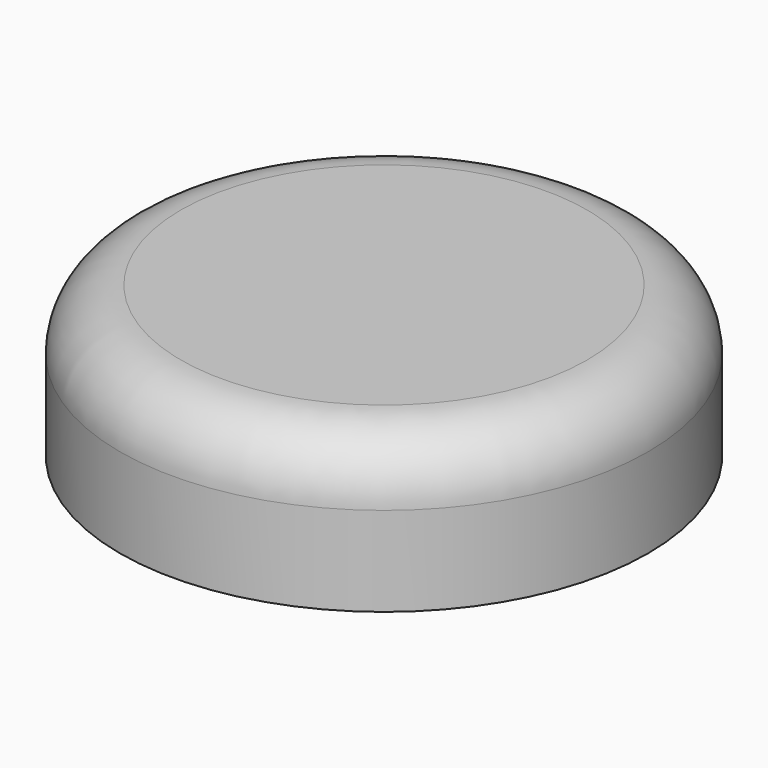
from build123d import *

# Parameters (mm, degrees)
F0_R     = 6.5
F1_DEPTH = 3.7
F2_R     = 1.5


# Not quite as in the source:
# - a feature of the source that left no trace in its solid (it failed there, or was rolled back) is left out


with BuildPart() as f1:
    # F0 (on Top) → F1 (new body)
    with BuildSketch(Plane.XY):
        Circle(F0_R)
    extrude(amount=F1_DEPTH)

    # F2
    f2_edges = [f1.edges().sort_by_distance(p)[0] for p in [
        (-6.5, 0, 3.7),
    ]]
    fillet(f2_edges, radius=F2_R)


solid = f1.part
